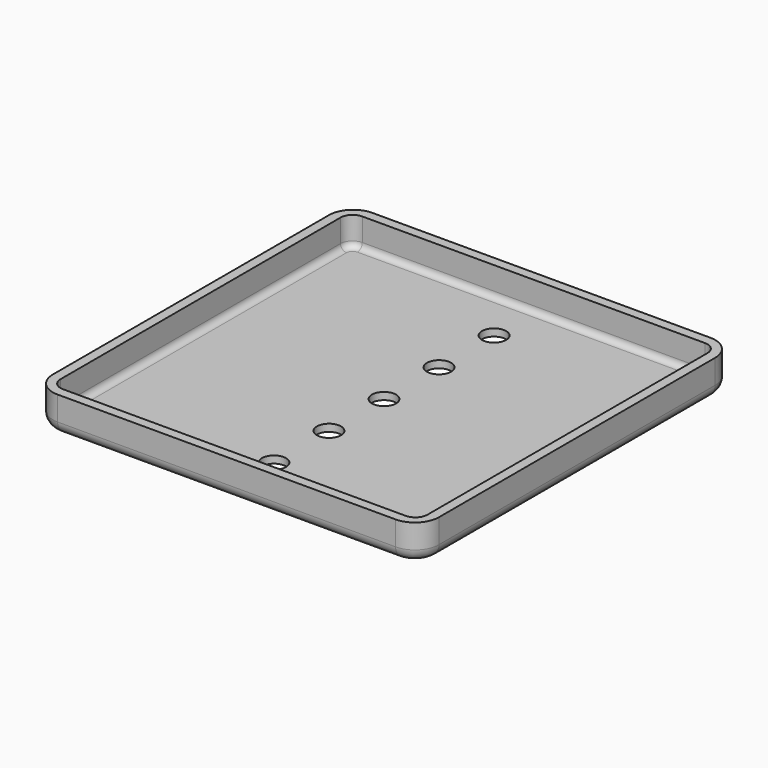
from build123d import *

# Parameters (mm, degrees)
F0_W         = 81.28
F0_H         = 82.804
F0_W_2       = 77.216
F0_H_2       = 78.74
F1_DEPTH     = 7.62
F2_DEPTH     = 1.524
F3_R         = 2.54
F4_R         = 1.27
F5_R         = 2.54
F6_DEPTH     = 25.4
F7_T1_DEPTH  = 20.32
F7_T4_ANGLE  = 90
F7_T6_ANGLE  = 90
F7_T8_ANGLE  = 90
F7_T10_ANGLE = 90


# Not quite as in the source:
# - a fillet or chamfer that OpenCascade refuses, or shapes differently, is made with other operations: its cross-section is extruded or revolved along the edge and cut away or added


with BuildPart() as f1:
    # F0 (on Top) → F1 (new body)
    with BuildSketch(Plane.XY):
        Rectangle(F0_W, F0_H)
        Rectangle(F0_W_2, F0_H_2, mode=Mode.SUBTRACT)
    extrude(amount=F1_DEPTH)

    # F0 (on Top) → F2 (join)
    with BuildSketch(Plane.XY):
        Rectangle(F0_W, F0_H)
        Rectangle(F0_W_2, F0_H_2, mode=Mode.SUBTRACT)
        Rectangle(F0_W_2, F0_H_2)
    extrude(amount=F2_DEPTH)

    # F3
    f3_edges = [f1.edges().sort_by_distance(p)[0] for p in [
        (-38.608, 39.37, 4.572),
        (38.608, 39.37, 4.572),
        (38.608, -39.37, 4.572),
        (-38.608, -39.37, 4.572),
        (0, 41.402, 0),
        (-40.64, 0, 0),
        (0, -41.402, 0),
        (40.64, 0, 0),
    ]]
    fillet(f3_edges, radius=F3_R)

    # F4
    f4_edges = [f1.edges().sort_by_distance(p)[0] for p in [
        (-38.608, 0, 1.524),
        (-37.864051, -38.626051, 1.524),
        (-37.864051, 38.626051, 1.524),
        (0, -39.37, 1.524),
        (0, 39.37, 1.524),
        (37.864051, -38.626051, 1.524),
        (37.864051, 38.626051, 1.524),
        (38.608, 0, 1.524),
    ]]
    fillet(f4_edges, radius=F4_R)

    # F5 (on face) → F6 (cut)
    with BuildSketch(Plane.XY.offset(1.524)):
        with Locations((0, 28.956)):
            Circle(F5_R)
        with Locations((0, 14.478)):
            Circle(F5_R)
        Circle(F5_R)
        with Locations((0, -14.478)):
            Circle(F5_R)
        with Locations((0, -28.956)):
            Circle(F5_R)
    extrude(amount=-F6_DEPTH, mode=Mode.SUBTRACT)

    # F7: fillet of radius 5.08 on 4 edges, made by hand

    # F7_s2 → F7_t1 (cut)
    with BuildSketch(Plane.XY):
        with BuildLine():
            ThreePointArc((35.56, -41.402), (39.1521024484, -39.9141024484), (40.64, -36.322))
            Line((40.64, -36.322), (40.64, -41.402))
            Line((40.64, -41.402), (35.56, -41.402))
        make_face()
        with BuildLine():
            ThreePointArc((35.56, 41.402), (39.1521024484, 39.9141024484), (40.64, 36.322))
            Line((40.64, 36.322), (40.64, 41.402))
            Line((40.64, 41.402), (35.56, 41.402))
        make_face()
        with BuildLine():
            ThreePointArc((-35.56, 41.402), (-39.1521024484, 39.9141024484), (-40.64, 36.322))
            Line((-40.64, 36.322), (-40.64, 41.402))
            Line((-40.64, 41.402), (-35.56, 41.402))
        make_face()
        with BuildLine():
            ThreePointArc((-40.64, -36.322), (-39.1521024484, -39.9141024484), (-35.56, -41.402))
            Line((-35.56, -41.402), (-40.64, -41.402))
            Line((-40.64, -41.402), (-40.64, -36.322))
        make_face()
    extrude(amount=F7_T1_DEPTH, mode=Mode.SUBTRACT)

    # F7_s3 → F7_t4 (revolve, cut)
    with BuildSketch(Plane.YZ.offset(-35.56)):
        with BuildLine():
            ThreePointArc((-38.862, 0), (-40.6580512242, 0.7439487758), (-41.402, 2.54))
            Line((-41.402, 2.54), (-41.402, 0))
            Line((-41.402, 0), (-38.862, 0))
        make_face()
    revolve(axis=Axis((-35.56, -36.322, 0), (0, 0, -1)), revolution_arc=F7_T4_ANGLE, mode=Mode.SUBTRACT)

    # F7_s5 → F7_t6 (revolve, cut)
    with BuildSketch(Plane.XZ.offset(-36.322)):
        with BuildLine():
            ThreePointArc((-38.1, 0), (-39.8960512242, 0.7439487758), (-40.64, 2.54))
            Line((-40.64, 2.54), (-40.64, 0))
            Line((-40.64, 0), (-38.1, 0))
        make_face()
    revolve(axis=Axis((-35.56, 36.322, 0), (0, 0, -1)), revolution_arc=F7_T6_ANGLE, mode=Mode.SUBTRACT)

    # F7_s7 → F7_t8 (revolve, cut)
    with BuildSketch(Plane.YZ.offset(35.56)):
        with BuildLine():
            ThreePointArc((38.862, 0), (40.6580512242, 0.7439487758), (41.402, 2.54))
            Line((41.402, 2.54), (41.402, 0))
            Line((41.402, 0), (38.862, 0))
        make_face()
    revolve(axis=Axis((35.56, 36.322, 0), (0, 0, -1)), revolution_arc=F7_T8_ANGLE, mode=Mode.SUBTRACT)

    # F7_s9 → F7_t10 (revolve, cut)
    with BuildSketch(Plane.XZ.offset(36.322)):
        with BuildLine():
            ThreePointArc((38.1, 0), (39.8960512242, 0.7439487758), (40.64, 2.54))
            Line((40.64, 2.54), (40.64, 0))
            Line((40.64, 0), (38.1, 0))
        make_face()
    revolve(axis=Axis((35.56, -36.322, 0), (0, 0, -1)), revolution_arc=F7_T10_ANGLE, mode=Mode.SUBTRACT)


solid = f1.part
